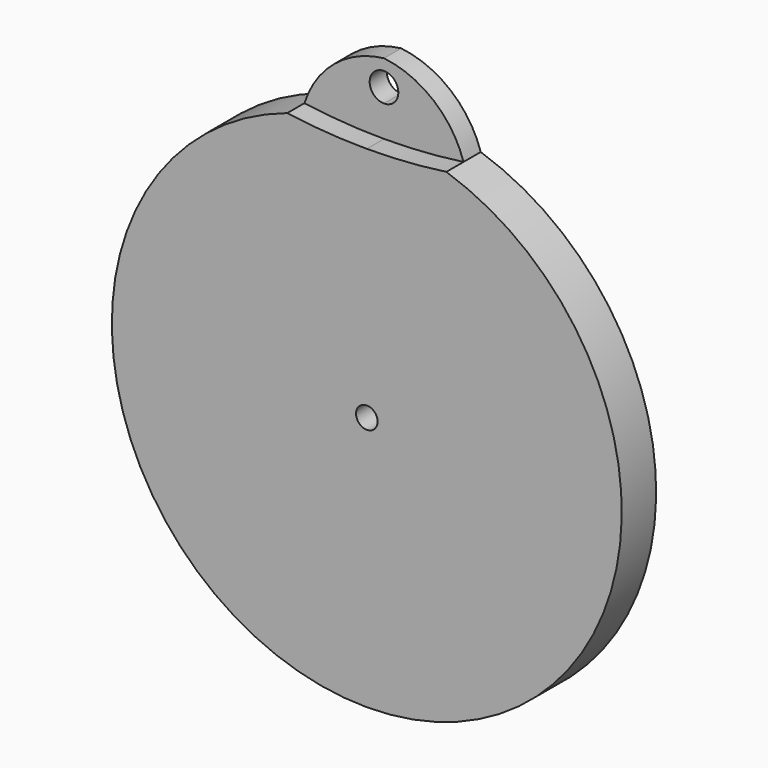
from build123d import *

# Parameters (mm, degrees)
F1_DEPTH = 3
F2_DEPTH = 6


# Not quite as in the source:
# - the program builds the solid bodies; features that only make, move or delete a surface that nothing else refers to are left out


with BuildPart() as f1:
    # F0 (on Front) → F1 (new body)
    with BuildSketch(Plane.XZ):
        with BuildLine():
            ThreePointArc((-36.2547188994, 42.8754752639), (-41.8166946482, 43.071513271), (-47.3510663807, 43.6586543583))
            ThreePointArc((-47.3510663807, 43.6586543583), (-36.2547188994, -25.6966625147), (-25.1583714182, 43.6586543583))
            ThreePointArc((-25.1583714182, 43.6586543583), (-30.6927431507, 43.071513271), (-36.2547188994, 42.8754752639))
        make_face()
        with BuildLine():
            ThreePointArc((-34.7547188994, 9.8686634646), (-37.3153790712, 8.8080032929), (-36.2547188994, 11.3686634646))
            ThreePointArc((-36.2547188994, 11.3686634646), (-35.1940587277, 10.9293236364), (-34.7547188994, 9.8686634646))
        make_face(mode=Mode.SUBTRACT)
        with BuildLine():
            ThreePointArc((-36.2547188994, 52.7826075633), (-43.1513282612, 49.8605681538), (-47.3510663807, 43.6586543583))
            ThreePointArc((-47.3510663807, 43.6586543583), (-41.8166946482, 43.071513271), (-36.2547188994, 42.8754752639))
            Line((-36.2547188994, 42.8754752639), (-36.2547188994, 47.2246634646))
            ThreePointArc((-36.2547188994, 47.2246634646), (-38.2547188994, 49.2246634646), (-36.2547188994, 51.2246634646))
            Line((-36.2547188994, 51.2246634646), (-36.2547188994, 52.7826075633))
        make_face()
        with BuildLine():
            ThreePointArc((-36.2547188994, 42.8754752639), (-30.6927431507, 43.071513271), (-25.1583714182, 43.6586543583))
            ThreePointArc((-25.1583714182, 43.6586543583), (-29.3581095377, 49.8605681538), (-36.2547188994, 52.7826075633))
            Line((-36.2547188994, 52.7826075633), (-36.2547188994, 51.2246634646))
            ThreePointArc((-36.2547188994, 51.2246634646), (-34.8405053371, 50.638877027), (-34.2547188994, 49.2246634646))
            ThreePointArc((-34.2547188994, 49.2246634646), (-34.8405053371, 47.8104499023), (-36.2547188994, 47.2246634646))
            Line((-36.2547188994, 47.2246634646), (-36.2547188994, 42.8754752639))
        make_face()
    extrude(amount=F1_DEPTH)

    # F0 (on Front) → F2 (join)
    with BuildSketch(Plane.XZ):
        with BuildLine():
            ThreePointArc((-36.2547188994, 42.8754752639), (-41.8166946482, 43.071513271), (-47.3510663807, 43.6586543583))
            ThreePointArc((-47.3510663807, 43.6586543583), (-36.2547188994, -25.6966625147), (-25.1583714182, 43.6586543583))
            ThreePointArc((-25.1583714182, 43.6586543583), (-30.6927431507, 43.071513271), (-36.2547188994, 42.8754752639))
        make_face()
        with BuildLine():
            ThreePointArc((-34.7547188994, 9.8686634646), (-37.3153790712, 8.8080032929), (-36.2547188994, 11.3686634646))
            ThreePointArc((-36.2547188994, 11.3686634646), (-35.1940587277, 10.9293236364), (-34.7547188994, 9.8686634646))
        make_face(mode=Mode.SUBTRACT)
    extrude(amount=F2_DEPTH)


solid = f1.part
